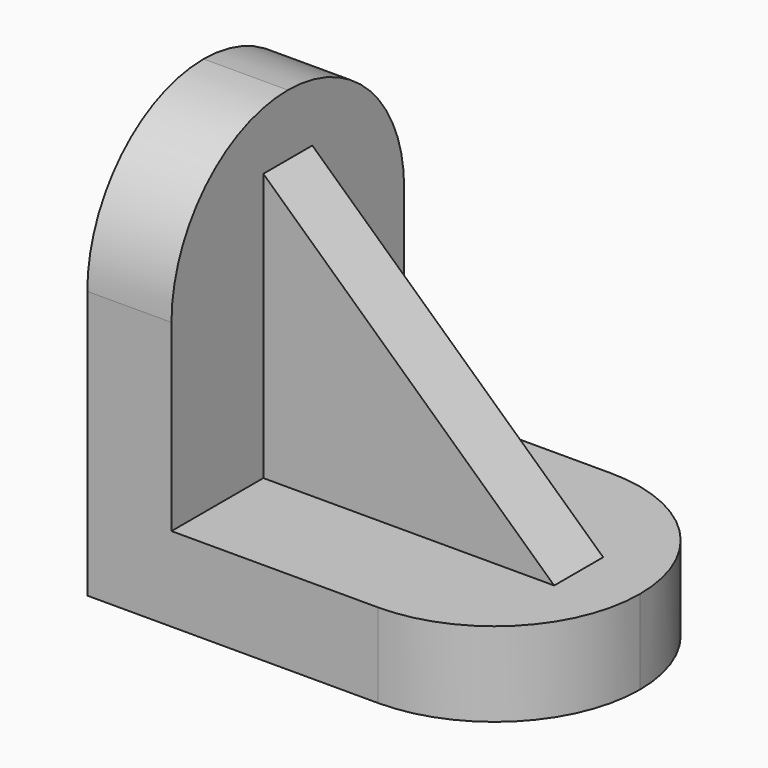
from build123d import *

# Parameters (mm, degrees)
F1_DEPTH = 19
F2_R     = 18.99999
F4_DEPTH = 4


# Not quite as in the source:
# - a fillet or chamfer is up to 0.001 mm smaller than in the source, because OpenCascade refuses the exact size


with BuildPart() as f1:
    # F0 (on Front) → F1 (new body, symmetric)
    with BuildSketch(Plane.XZ):
        Polygon((0, 54), (0, 0), (57, 0), (57, 11), (11, 11), (11, 54), align=None)
    extrude(amount=F1_DEPTH, both=True)

    # F2 (radius 19 in the source; OpenCascade refuses exactly that, so slightly less here)
    f2_edges = [f1.edges().sort_by_distance(p)[0] for p in [
        (5.5, -19, 54),
        (5.5, 19, 54),
        (57, -19, 5.5),
        (57, 19, 5.5),
    ]]
    fillet(f2_edges, radius=F2_R)

    # F3 (on Front) → F4 (join, symmetric)
    with BuildSketch(Plane.XZ):
        Polygon((49, 11), (11, 46), (11, 35), (11, 11), (38, 11), align=None)
    extrude(amount=F4_DEPTH, both=True)


solid = f1.part
